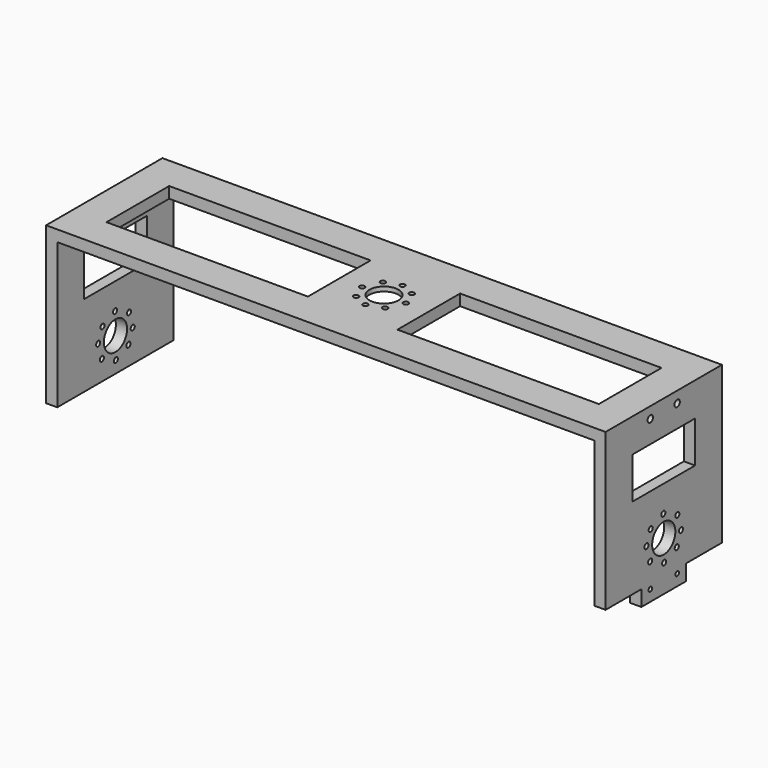
from build123d import *

# Parameters (mm, degrees)
F0_W           = 5
F0_H           = 65
F0_W_2         = 240
F1_DEPTH       = 5
F2_W           = 5
F2_H           = 65
F3_DEPTH       = 65
F4_R           = 6.477
F5_DEPTH       = 250.001
F6_R           = 6.477
F7_DEPTH       = 25.4
F8_W           = 90
F8_H           = 35
F9_DEPTH       = 25.4
F10_W          = 35
F10_H          = 18.523
F11_DEPTH      = 245.001
F11_DEPTH_BACK = 25.4
F12_R          = 1.5
F13_DEPTH      = 25.4
F12_W          = 25
F12_H          = 7
F12_R_2        = 1
F14_DEPTH      = 5
F15_R          = 13.335
F15_R_2        = 6.477
F16_DEPTH      = 3
F17_R          = 1.143
F18_DEPTH      = 2.001
F19_R          = 1.143
F20_DEPTH      = 250.001


# Not quite as in the source:
# - a feature names something its author has since deleted; it is built from what else it names


with BuildPart() as f1:
    # F0 (on Top) → F1 (new body)
    with BuildSketch(Plane.XY):
        with Locations((-114.2006202787, -15.5218991437)):
            Rectangle(F0_W, F0_H)
        with Locations((130.7993797213, -15.5218991437)):
            Rectangle(F0_W, F0_H)
        with Locations((8.2993797213, -15.5218991437)):
            Rectangle(F0_W_2, F0_H)
    extrude(amount=F1_DEPTH)

    # F2 (on face) → F3 (join)
    with BuildSketch(Plane(origin=(0, 0, 0), x_dir=(1, 0, 0), z_dir=(0, 0, -1))):
        with Locations((-114.2006202787, 15.5218991437)):
            Rectangle(F2_W, F2_H)
        with Locations((130.7993797213, 15.5218991437)):
            Rectangle(F2_W, F2_H)
    extrude(amount=F3_DEPTH)

    # F4 (on face) → F5 (cut, through all)
    with BuildSketch(Plane.YZ.offset(133.2993797213)):
        with Locations((-15.5218991437, -50)):
            Circle(F4_R)
    extrude(amount=-F5_DEPTH, mode=Mode.SUBTRACT)

    # F6 (on face) → F7 (cut)
    with BuildSketch(Plane(origin=(0, 0, 0), x_dir=(1, 0, 0), z_dir=(0, 0, -1))):
        with Locations((8.2993797213, 15.5218991437)):
            Circle(F6_R)
    extrude(amount=-F7_DEPTH, mode=Mode.SUBTRACT)

    # F8 (on face) → F9 (cut)
    with BuildSketch(Plane(origin=(0, 0, 0), x_dir=(1, 0, 0), z_dir=(0, 0, -1))):
        with Locations((-56.7006202787, 15.5218991437)):
            Rectangle(F8_W, F8_H)
        with Locations((73.2993797213, 15.5218991437)):
            Rectangle(F8_W, F8_H)
    extrude(amount=-F9_DEPTH, mode=Mode.SUBTRACT)

    # F10 (on face) → F11 (cut, two sides)
    with BuildSketch(Plane.YZ.offset(-111.7006202787)) as f11_sk:
        with Locations((-15.5218991437, -19.2615)):
            Rectangle(F10_W, F10_H)
    extrude(amount=F11_DEPTH, mode=Mode.SUBTRACT)
    extrude(f11_sk.sketch, amount=-F11_DEPTH_BACK, mode=Mode.SUBTRACT)

    # F12 (on face) → F13 (cut)
    with BuildSketch(Plane.YZ.offset(133.2993797213)):
        with Locations((-23.0218991437, 0)):
            Circle(F12_R)
        with Locations((-8.0218991437, 0)):
            Circle(F12_R)
    extrude(amount=-F13_DEPTH, mode=Mode.SUBTRACT)

    # F12 (on face) → F14 (join, through all)
    with BuildSketch(Plane.YZ.offset(133.2993797213)):
        with Locations((-15.5218991437, -68.5)):
            Rectangle(F12_W, F12_H)
        with Locations((-23.0218991437, -67)):
            Circle(F12_R_2, mode=Mode.SUBTRACT)
        with Locations((-8.0218991437, -67)):
            Circle(F12_R_2, mode=Mode.SUBTRACT)
    extrude(amount=-F14_DEPTH)

    # F15 (on face) → F16 (cut)
    with BuildSketch(Plane(origin=(0, 0, 0), x_dir=(1, 0, 0), z_dir=(0, 0, -1))):
        with Locations((8.2993797213, 15.5218991437)):
            Circle(F15_R)
        with Locations((8.2993797213, 15.5218991437)):
            Circle(F15_R_2, mode=Mode.SUBTRACT)
    extrude(amount=-F16_DEPTH, mode=Mode.SUBTRACT)

    # F17 (on face) → F18 (cut, through all)
    with BuildSketch(Plane(origin=(0, 0, 3), x_dir=(1, 0, 0), z_dir=(0, 0, -1))):
        with Locations((14.6909433031, 22.9230312179)):
            Circle(F17_R)
        with Locations((18.0783797213, 15.5218991437)):
            Circle(F17_R)
        with Locations((15.2324973507, 8.6286974185)):
            Circle(F17_R)
        with Locations((8.8073272824, 5.7887949694)):
            Circle(F17_R)
        with Locations((1.9078161395, 8.1207670695)):
            Circle(F17_R)
        with Locations((-1.4796202787, 15.5218991437)):
            Circle(F17_R)
        with Locations((1.3662620919, 22.415100869)):
            Circle(F17_R)
        with Locations((7.7914321602, 25.2550033181)):
            Circle(F17_R)
    extrude(amount=-F18_DEPTH, mode=Mode.SUBTRACT)

    # F19 (on face) → F20 (cut, through all)
    with BuildSketch(Plane(origin=(-116.7006202787, 0, 0), x_dir=(0, -1, 0), z_dir=(-1, 0, 0))):
        with Locations((15.765312519, -40.2836638916)):
            Circle(F19_R)
        with Locations((25.1764905212, -49.2415353535)):
            Circle(F19_R)
        with Locations((23.1101417116, -56.0547046433)):
            Circle(F19_R)
        with Locations((15.2784857684, -59.7163361084)):
            Circle(F19_R)
        with Locations((8.2459797528, -56.5320689682)):
            Circle(F19_R)
        with Locations((5.8673077662, -50.7584646465)):
            Circle(F19_R)
        with Locations((7.9336565759, -43.9452953567)):
            Circle(F19_R)
        with Locations((22.7978185346, -43.4679310318)):
            Circle(F19_R)
    extrude(amount=-F20_DEPTH, mode=Mode.SUBTRACT)


solid = f1.part
